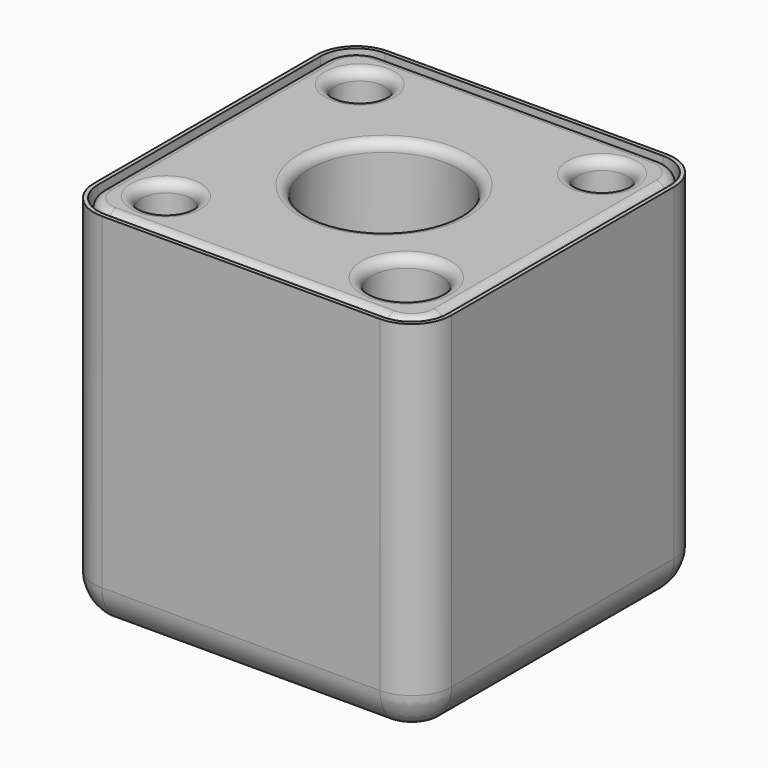
from build123d import *

# Parameters (mm, degrees)
F0_W      = 180
F0_H      = 180
F1_DEPTH  = 180
F2_R      = 20
F3_SIZE   = 7
F4_R      = 20
F5_T      = -2
F7_DEPTH  = 50
F8_R      = 37.5
F9_DEPTH  = 180.0010001
F10_R     = 37.5
F10_R_2   = 1.5
F11_DEPTH = 2
F12_R     = 12.5
F13_DEPTH = 20
F14_R     = 17.5
F15_DEPTH = 180.0010001
F16_R     = 5
F17_R     = 0.99999
F18_SIZE  = 7
F19_R     = 20


# Not quite as in the source:
# - a fillet or chamfer is up to 0.001 mm smaller than in the source, because OpenCascade refuses the exact size


with BuildPart() as f1:
    # F0 (on Top) → F1 (new body)
    with BuildSketch(Plane.XY):
        Rectangle(F0_W, F0_H)
    extrude(amount=F1_DEPTH)

    # F2
    f2_edges = [f1.edges().sort_by_distance(p)[0] for p in [
        (90, -90, 90),
        (-90, -90, 90),
        (90, 90, 90),
        (-90, 90, 90),
    ]]
    fillet(f2_edges, radius=F2_R)

    # F3
    f3_edges = [f1.edges().sort_by_distance(p)[0] for p in [
        (0, 90, 0),
        (84.142136, 84.142136, 0),
        (-84.142136, 84.142136, 0),
        (90, 0, 0),
        (-90, 0, 0),
        (84.142136, -84.142136, 0),
        (-84.142136, -84.142136, 0),
        (0, -90, 0),
    ]]
    chamfer(f3_edges, length=F3_SIZE)

    # F4
    f4_edges = [f1.edges().sort_by_distance(p)[0] for p in [
        (-90, 0, 7),
    ]]
    fillet(f4_edges, radius=F4_R)

    # F5
    f5_openings = [f1.faces().sort_by_distance(p)[0] for p in [
        (0, 0, 180),
    ]]
    offset(amount=F5_T, openings=f5_openings)


with BuildPart() as f7:
    # F6 (on face) → F7 (new body)
    with BuildSketch(Plane.XY.offset(180)):
        with BuildLine():
            ThreePointArc((-86, -70), (-81.313708499, -81.313708499), (-70, -86))
            Line((-70, -86), (70, -86))
            ThreePointArc((70, -86), (81.313708499, -81.313708499), (86, -70))
            Line((86, -70), (86, 70))
            ThreePointArc((86, 70), (81.313708499, 81.313708499), (70, 86))
            Line((70, 86), (-70, 86))
            ThreePointArc((-70, 86), (-81.313708499, 81.313708499), (-86, 70))
            Line((-86, 70), (-86, -70))
        make_face()
    extrude(amount=-F7_DEPTH)

    # F8 (on face) → F9 (cut, through all)
    with BuildSketch(Plane.XY.offset(180)):
        Circle(F8_R)
    extrude(amount=-F9_DEPTH, mode=Mode.SUBTRACT)

    # F10 (on face) → F11 (join)
    with BuildSketch(Plane(origin=(0, 0, 130), x_dir=(1, 0, 0), z_dir=(0, 0, -1))):
        Circle(F10_R)
        with Locations((-22.2943447643, -20.0739181908)):
            Circle(F10_R_2, mode=Mode.SUBTRACT)
        with Locations((-6.2373507245, -29.344428022)):
            Circle(F10_R_2, mode=Mode.SUBTRACT)
        with Locations((-17.6335575688, -24.2705098312)):
            Circle(F10_R_2, mode=Mode.SUBTRACT)
        with Locations((-12.2020992923, -27.4063637293)):
            Circle(F10_R_2, mode=Mode.SUBTRACT)
        with Locations((-12, -20.7846096908)):
            Circle(F10_R_2, mode=Mode.SUBTRACT)
        with Locations((-6.2116570825, -23.1822198309)):
            Circle(F10_R_2, mode=Mode.SUBTRACT)
        with Locations((-25.9807621135, -15)):
            Circle(F10_R_2, mode=Mode.SUBTRACT)
        with Locations((-20.7846096908, -12)):
            Circle(F10_R_2, mode=Mode.SUBTRACT)
        with Locations((-28.5316954889, -9.2705098312)):
            Circle(F10_R_2, mode=Mode.SUBTRACT)
        with Locations((-29.835656861, -3.135853898)):
            Circle(F10_R_2, mode=Mode.SUBTRACT)
        with Locations((-23.1822198309, -6.2116570825)):
            Circle(F10_R_2, mode=Mode.SUBTRACT)
        with Locations((-16.9705627485, -16.9705627485)):
            Circle(F10_R_2, mode=Mode.SUBTRACT)
        with Locations((-11.5701769744, -13.7887999761)):
            Circle(F10_R_2, mode=Mode.SUBTRACT)
        with Locations((-6.1563625799, -16.9144671741)):
            Circle(F10_R_2, mode=Mode.SUBTRACT)
        with Locations((-6, -10.3923048454)):
            Circle(F10_R_2, mode=Mode.SUBTRACT)
        with Locations((-15.5884572681, -9)):
            Circle(F10_R_2, mode=Mode.SUBTRACT)
        with Locations((-10.3923048454, -6)):
            Circle(F10_R_2, mode=Mode.SUBTRACT)
        with Locations((-17.7265395542, -3.125667198)):
            Circle(F10_R_2, mode=Mode.SUBTRACT)
        with Locations((-5.1961524227, -3)):
            Circle(F10_R_2, mode=Mode.SUBTRACT)
        with Locations((0, -30)):
            Circle(F10_R_2, mode=Mode.SUBTRACT)
        with Locations((6.2373507245, -29.344428022)):
            Circle(F10_R_2, mode=Mode.SUBTRACT)
        with Locations((0, -24)):
            Circle(F10_R_2, mode=Mode.SUBTRACT)
        with Locations((6.2116570825, -23.1822198309)):
            Circle(F10_R_2, mode=Mode.SUBTRACT)
        with Locations((12.2020992923, -27.4063637293)):
            Circle(F10_R_2, mode=Mode.SUBTRACT)
        with Locations((17.6335575688, -24.2705098312)):
            Circle(F10_R_2, mode=Mode.SUBTRACT)
        with Locations((12, -20.7846096908)):
            Circle(F10_R_2, mode=Mode.SUBTRACT)
        with Locations((22.2943447643, -20.0739181908)):
            Circle(F10_R_2, mode=Mode.SUBTRACT)
        with Locations((0, -18)):
            Circle(F10_R_2, mode=Mode.SUBTRACT)
        with Locations((6.1563625799, -16.9144671741)):
            Circle(F10_R_2, mode=Mode.SUBTRACT)
        with Locations((0, -12)):
            Circle(F10_R_2, mode=Mode.SUBTRACT)
        with Locations((6, -10.3923048454)):
            Circle(F10_R_2, mode=Mode.SUBTRACT)
        with Locations((16.9705627485, -16.9705627485)):
            Circle(F10_R_2, mode=Mode.SUBTRACT)
        with Locations((11.5701769744, -13.7887999761)):
            Circle(F10_R_2, mode=Mode.SUBTRACT)
        with Locations((0, -6)):
            Circle(F10_R_2, mode=Mode.SUBTRACT)
        with Locations((5.1961524227, -3)):
            Circle(F10_R_2, mode=Mode.SUBTRACT)
        with Locations((10.3923048454, -6)):
            Circle(F10_R_2, mode=Mode.SUBTRACT)
        with Locations((15.5884572681, -9)):
            Circle(F10_R_2, mode=Mode.SUBTRACT)
        with Locations((17.7265395542, -3.125667198)):
            Circle(F10_R_2, mode=Mode.SUBTRACT)
        with Locations((25.9807621135, -15)):
            Circle(F10_R_2, mode=Mode.SUBTRACT)
        with Locations((20.7846096908, -12)):
            Circle(F10_R_2, mode=Mode.SUBTRACT)
        with Locations((23.1822198309, -6.2116570825)):
            Circle(F10_R_2, mode=Mode.SUBTRACT)
        with Locations((28.5316954889, -9.2705098312)):
            Circle(F10_R_2, mode=Mode.SUBTRACT)
        with Locations((29.835656861, -3.135853898)):
            Circle(F10_R_2, mode=Mode.SUBTRACT)
        with Locations((-29.835656861, 3.135853898)):
            Circle(F10_R_2, mode=Mode.SUBTRACT)
        with Locations((-28.5316954889, 9.2705098312)):
            Circle(F10_R_2, mode=Mode.SUBTRACT)
        with Locations((-24, 0)):
            Circle(F10_R_2, mode=Mode.SUBTRACT)
        with Locations((-23.1822198309, 6.2116570825)):
            Circle(F10_R_2, mode=Mode.SUBTRACT)
        with Locations((-20.7846096908, 12)):
            Circle(F10_R_2, mode=Mode.SUBTRACT)
        with Locations((-25.9807621135, 15)):
            Circle(F10_R_2, mode=Mode.SUBTRACT)
        with Locations((-17.7265395542, 3.125667198)):
            Circle(F10_R_2, mode=Mode.SUBTRACT)
        with Locations((-12, 0)):
            Circle(F10_R_2, mode=Mode.SUBTRACT)
        with Locations((-15.5884572681, 9)):
            Circle(F10_R_2, mode=Mode.SUBTRACT)
        with Locations((-10.3923048454, 6)):
            Circle(F10_R_2, mode=Mode.SUBTRACT)
        with Locations((-5.1961524227, 3)):
            Circle(F10_R_2, mode=Mode.SUBTRACT)
        with Locations((-11.5701769744, 13.7887999761)):
            Circle(F10_R_2, mode=Mode.SUBTRACT)
        with Locations((-16.9705627485, 16.9705627485)):
            Circle(F10_R_2, mode=Mode.SUBTRACT)
        with Locations((-6, 10.3923048454)):
            Circle(F10_R_2, mode=Mode.SUBTRACT)
        with Locations((-6.1563625799, 16.9144671741)):
            Circle(F10_R_2, mode=Mode.SUBTRACT)
        with Locations((-22.2943447643, 20.0739181908)):
            Circle(F10_R_2, mode=Mode.SUBTRACT)
        with Locations((-12, 20.7846096908)):
            Circle(F10_R_2, mode=Mode.SUBTRACT)
        with Locations((-17.6335575688, 24.2705098312)):
            Circle(F10_R_2, mode=Mode.SUBTRACT)
        with Locations((-12.2020992923, 27.4063637293)):
            Circle(F10_R_2, mode=Mode.SUBTRACT)
        with Locations((-6.2116570825, 23.1822198309)):
            Circle(F10_R_2, mode=Mode.SUBTRACT)
        with Locations((-6.2373507245, 29.344428022)):
            Circle(F10_R_2, mode=Mode.SUBTRACT)
        Circle(F10_R_2, mode=Mode.SUBTRACT)
        with Locations((5.1961524227, 3)):
            Circle(F10_R_2, mode=Mode.SUBTRACT)
        with Locations((0, 6)):
            Circle(F10_R_2, mode=Mode.SUBTRACT)
        with Locations((12, 0)):
            Circle(F10_R_2, mode=Mode.SUBTRACT)
        with Locations((17.7265395542, 3.125667198)):
            Circle(F10_R_2, mode=Mode.SUBTRACT)
        with Locations((10.3923048454, 6)):
            Circle(F10_R_2, mode=Mode.SUBTRACT)
        with Locations((15.5884572681, 9)):
            Circle(F10_R_2, mode=Mode.SUBTRACT)
        with Locations((0, 12)):
            Circle(F10_R_2, mode=Mode.SUBTRACT)
        with Locations((6, 10.3923048454)):
            Circle(F10_R_2, mode=Mode.SUBTRACT)
        with Locations((0, 18)):
            Circle(F10_R_2, mode=Mode.SUBTRACT)
        with Locations((6.1563625799, 16.9144671741)):
            Circle(F10_R_2, mode=Mode.SUBTRACT)
        with Locations((11.5701769744, 13.7887999761)):
            Circle(F10_R_2, mode=Mode.SUBTRACT)
        with Locations((16.9705627485, 16.9705627485)):
            Circle(F10_R_2, mode=Mode.SUBTRACT)
        with Locations((24, 0)):
            Circle(F10_R_2, mode=Mode.SUBTRACT)
        with Locations((23.1822198309, 6.2116570825)):
            Circle(F10_R_2, mode=Mode.SUBTRACT)
        with Locations((29.835656861, 3.135853898)):
            Circle(F10_R_2, mode=Mode.SUBTRACT)
        with Locations((28.5316954889, 9.2705098312)):
            Circle(F10_R_2, mode=Mode.SUBTRACT)
        with Locations((20.7846096908, 12)):
            Circle(F10_R_2, mode=Mode.SUBTRACT)
        with Locations((25.9807621135, 15)):
            Circle(F10_R_2, mode=Mode.SUBTRACT)
        with Locations((6.2116570825, 23.1822198309)):
            Circle(F10_R_2, mode=Mode.SUBTRACT)
        with Locations((0, 24)):
            Circle(F10_R_2, mode=Mode.SUBTRACT)
        with Locations((12, 20.7846096908)):
            Circle(F10_R_2, mode=Mode.SUBTRACT)
        with Locations((12.2020992923, 27.4063637293)):
            Circle(F10_R_2, mode=Mode.SUBTRACT)
        with Locations((17.6335575688, 24.2705098312)):
            Circle(F10_R_2, mode=Mode.SUBTRACT)
        with Locations((0, 30)):
            Circle(F10_R_2, mode=Mode.SUBTRACT)
        with Locations((6.2373507245, 29.344428022)):
            Circle(F10_R_2, mode=Mode.SUBTRACT)
        with Locations((22.2943447643, 20.0739181908)):
            Circle(F10_R_2, mode=Mode.SUBTRACT)
    extrude(amount=-F11_DEPTH)

    # F12 (on face) → F13 (cut)
    with BuildSketch(Plane.XY.offset(180)):
        with Locations((-61, -61)):
            Circle(F12_R)
        with Locations((-61, 61)):
            Circle(F12_R)
        with Locations((61, 61)):
            Circle(F12_R)
    extrude(amount=-F13_DEPTH, mode=Mode.SUBTRACT)

    # F14 (on face) → F15 (cut, through all)
    with BuildSketch(Plane.XY.offset(180)):
        with Locations((56, -56)):
            Circle(F14_R)
    extrude(amount=-F15_DEPTH, mode=Mode.SUBTRACT)

    # F16
    f16_edges = [f7.edges().sort_by_distance(p)[0] for p in [
        (-81.313708, 81.313708, 180),
        (0, 86, 180),
        (-86, 0, 180),
        (81.313708, 81.313708, 180),
        (-81.313708, -81.313708, 180),
        (86, 0, 180),
        (0, -86, 180),
        (81.313708, -81.313708, 180),
        (-73.5, -61, 180),
        (38.5, -56, 180),
        (-73.5, 61, 180),
        (-37.5, 0, 180),
        (48.5, 61, 180),
        (-37.5, 0, 132),
    ]]
    fillet(f16_edges, radius=F16_R)

    # F17 (radius 1 in the source; OpenCascade refuses exactly that, so slightly less here)
    f17_edges = [f7.edges().sort_by_distance(p)[0] for p in [
        (-32.5, 0, 132),
        (-23.794345, 20.073918, 132),
        (-7.737351, 29.344428, 132),
        (-19.133558, 24.27051, 132),
        (-13.702099, 27.406364, 132),
        (-13.5, 20.78461, 132),
        (-7.711657, 23.18222, 132),
        (-27.480762, 15, 132),
        (-22.28461, 12, 132),
        (-30.031695, 9.27051, 132),
        (-31.335657, 3.135854, 132),
        (-24.68222, 6.211657, 132),
        (-18.470563, 16.970563, 132),
        (-13.070177, 13.7888, 132),
        (-7.656363, 16.914467, 132),
        (-7.5, 10.392305, 132),
        (-17.088457, 9, 132),
        (-11.892305, 6, 132),
        (-19.22654, 3.125667, 132),
        (-6.696152, 3, 132),
        (-1.5, 30, 132),
        (4.737351, 29.344428, 132),
        (-1.5, 24, 132),
        (4.711657, 23.18222, 132),
        (10.702099, 27.406364, 132),
        (16.133558, 24.27051, 132),
        (10.5, 20.78461, 132),
        (20.794345, 20.073918, 132),
        (-1.5, 18, 132),
        (4.656363, 16.914467, 132),
        (-1.5, 12, 132),
        (4.5, 10.392305, 132),
        (15.470563, 16.970563, 132),
        (10.070177, 13.7888, 132),
        (-1.5, 6, 132),
        (3.696152, 3, 132),
        (8.892305, 6, 132),
        (14.088457, 9, 132),
        (16.22654, 3.125667, 132),
        (24.480762, 15, 132),
        (19.28461, 12, 132),
        (21.68222, 6.211657, 132),
        (27.031695, 9.27051, 132),
        (28.335657, 3.135854, 132),
        (-31.335657, -3.135854, 132),
        (-30.031695, -9.27051, 132),
        (-25.5, 0, 132),
        (-24.68222, -6.211657, 132),
        (-22.28461, -12, 132),
        (-27.480762, -15, 132),
        (-19.22654, -3.125667, 132),
        (-13.5, 0, 132),
        (-17.088457, -9, 132),
        (-11.892305, -6, 132),
        (-6.696152, -3, 132),
        (-13.070177, -13.7888, 132),
        (-18.470563, -16.970563, 132),
        (-7.5, -10.392305, 132),
        (-7.656363, -16.914467, 132),
        (-23.794345, -20.073918, 132),
        (-13.5, -20.78461, 132),
        (-19.133558, -24.27051, 132),
        (-13.702099, -27.406364, 132),
        (-7.711657, -23.18222, 132),
        (-7.737351, -29.344428, 132),
        (-1.5, 0, 132),
        (3.696152, -3, 132),
        (-1.5, -6, 132),
        (10.5, 0, 132),
        (16.22654, -3.125667, 132),
        (8.892305, -6, 132),
        (14.088457, -9, 132),
        (-1.5, -12, 132),
        (4.5, -10.392305, 132),
        (-1.5, -18, 132),
        (4.656363, -16.914467, 132),
        (10.070177, -13.7888, 132),
        (15.470563, -16.970563, 132),
        (22.5, 0, 132),
        (21.68222, -6.211657, 132),
        (28.335657, -3.135854, 132),
        (27.031695, -9.27051, 132),
        (19.28461, -12, 132),
        (24.480762, -15, 132),
        (4.711657, -23.18222, 132),
        (-1.5, -24, 132),
        (10.5, -20.78461, 132),
        (10.702099, -27.406364, 132),
        (16.133558, -24.27051, 132),
        (-1.5, -30, 132),
        (4.737351, -29.344428, 132),
        (20.794345, -20.073918, 132),
    ]]
    fillet(f17_edges, radius=F17_R)

    # F18
    f18_edges = [f7.edges().sort_by_distance(p)[0] for p in [
        (0, -86, 130),
    ]]
    chamfer(f18_edges, length=F18_SIZE)

    # F19
    f19_edges = [f7.edges().sort_by_distance(p)[0] for p in [
        (0, -86, 137),
        (-81.313708, -81.313708, 137),
        (81.313708, -81.313708, 137),
        (-86, 0, 137),
        (86, 0, 137),
        (-81.313708, 81.313708, 137),
        (81.313708, 81.313708, 137),
        (0, 86, 137),
    ]]
    fillet(f19_edges, radius=F19_R)


solid = Compound([f1.part, f7.part])
